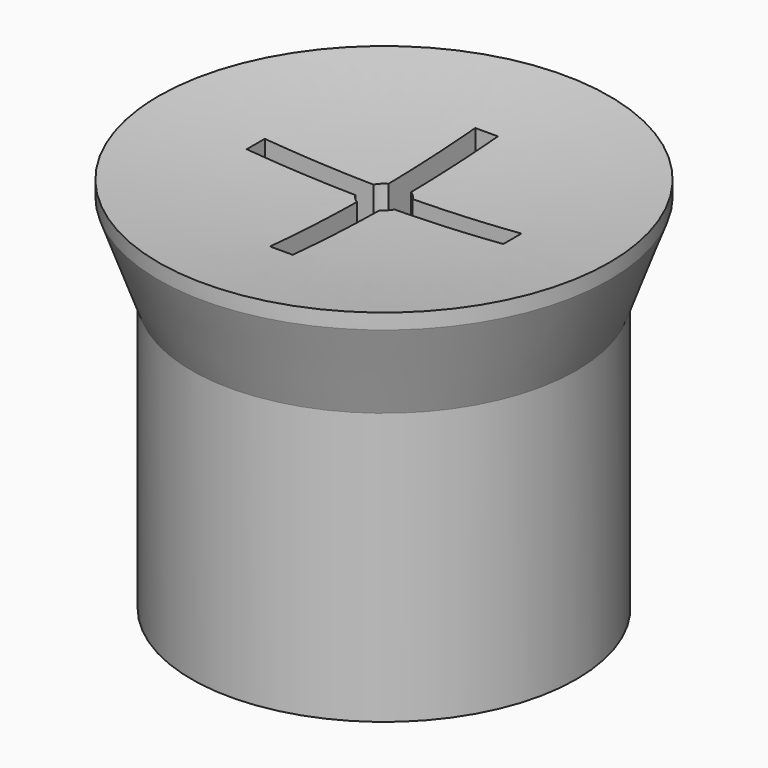
from build123d import *

# Parameters (mm, degrees)
F0_R      = 10.795
F1_DEPTH  = 15.24
F1_FACE_R = 10.795
F2_DEPTH  = 5.08
F2_TAPER  = -20
F3_DEPTH  = 1.016
F5_DEPTH  = 6.0706


with BuildPart() as f1:
    # F0 (on Top) → F1 (new body)
    with BuildSketch(Plane.XY):
        Circle(F0_R)
    extrude(amount=F1_DEPTH)

    # F1_face (on face) → F2 (join)
    with BuildSketch(Plane.XY.offset(15.24)):
        Circle(F1_FACE_R)
    extrude(amount=F2_DEPTH, taper=F2_TAPER)

    # F3 (add): a face of the model
    f3_faces = [f1.faces().sort_by_distance(p)[0] for p in [
        (0, 0, 20.32),
    ]]
    extrude(f3_faces, amount=F3_DEPTH)

    # F4 (on face) → F5 (cut)
    with BuildSketch(Plane.XY.offset(21.336)):
        with BuildLine():
            Line((0.635, 7.1958522628), (-0.635, 7.1958522628))
            Line((-0.635, 7.1958522628), (-0.635, 1.0998522628))
            ThreePointArc((-0.635, 1.0998522628), (-0.8980256121, 0.8980256121), (-1.0998522628, 0.635))
            Line((-1.0998522628, 0.635), (-7.1958522628, 0.635))
            Line((-7.1958522628, 0.635), (-7.1958522628, -0.635))
            Line((-7.1958522628, -0.635), (-1.0998522628, -0.635))
            ThreePointArc((-1.0998522628, -0.635), (-0.8980256121, -0.8980256121), (-0.635, -1.0998522628))
            Line((-0.635, -1.0998522628), (-0.635, -7.1958522628))
            Line((-0.635, -7.1958522628), (0.635, -7.1958522628))
            Line((0.635, -7.1958522628), (0.635, -1.0998522628))
            ThreePointArc((0.635, -1.0998522628), (0.8980256121, -0.8980256121), (1.0998522628, -0.635))
            Line((1.0998522628, -0.635), (7.1958522628, -0.635))
            Line((7.1958522628, -0.635), (7.1958522628, 0.635))
            Line((7.1958522628, 0.635), (1.0998522628, 0.635))
            ThreePointArc((1.0998522628, 0.635), (0.8980256121, 0.8980256121), (0.635, 1.0998522628))
            Line((0.635, 1.0998522628), (0.635, 7.1958522628))
        make_face()
    extrude(amount=-F5_DEPTH, mode=Mode.SUBTRACT)

    # F6 (on Front) → F7 (revolve, cut)
    with BuildSketch(Plane.XZ):
        with BuildLine():
            ThreePointArc((0, 201.9231468439), (-90.8144451678, 111.1087016761), (0, 20.2942565084))
            Line((0, 20.2942565084), (0, 201.9231468439))
        make_face()
    revolve(axis=Axis((0, 0, 111.1087016761), (0, 0, 1)), mode=Mode.SUBTRACT)


solid = f1.part
